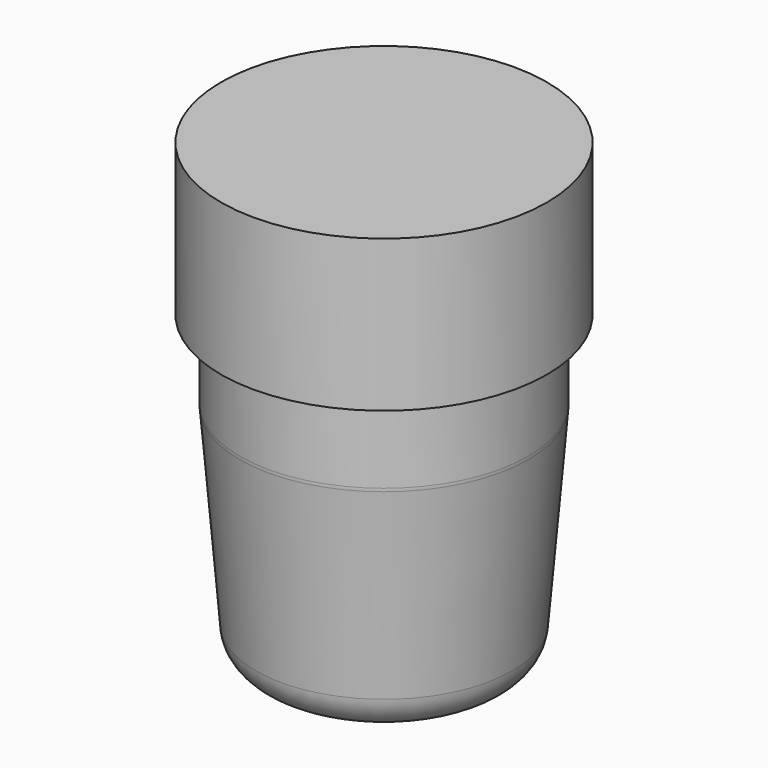
from build123d import *

# Parameters (mm, degrees)
F0_R     = 21.5
F1_DEPTH = 20
F2_R     = 19.0313090647
F3_DEPTH = 0.5
F4_R     = 19.0313090647
F5_DEPTH = 40


# Not quite as in the source:
# - a fillet or chamfer that OpenCascade refuses, or shapes differently, is made with other operations: its cross-section is extruded or revolved along the edge and cut away or added


with BuildPart() as f1:
    # F0 (on Top) → F1 (new body)
    with BuildSketch(Plane.XY):
        Circle(F0_R)
    extrude(amount=F1_DEPTH)

    # F2 (on face) → F3 (join)
    with BuildSketch(Plane(origin=(0, 0, 0), x_dir=(1, 0, 0), z_dir=(0, 0, -1))):
        Circle(F2_R)
    extrude(amount=F3_DEPTH)

    # F4 (on face) → F5 (join)
    with BuildSketch(Plane(origin=(0, 0, -0.5), x_dir=(1, 0, 0), z_dir=(0, 0, -1))):
        Circle(F4_R)
    extrude(amount=F5_DEPTH)

    # F6: chamfer of 2.5 x 30 on 1 edges, made by hand

    # F6_s1 → F6_t2 (revolve, cut)
    with BuildSketch(Plane.XZ):
        Polygon((19.0313090647, -10.5), (16.5313090647, -40.5), (19.0313090647, -40.5), align=None)
    revolve(axis=Axis((0, 0, -40.5), (0, 0, -1)), mode=Mode.SUBTRACT)

    # F7: fillet of radius 5 on 2 edges, made by hand

    # F7_s1 → F7_t2 (revolve, cut)
    with BuildSketch(Plane.XZ):
        with BuildLine():
            ThreePointArc((16.9133734481, -35.9152273993), (15.3161921018, -39.1794114337), (11.9306446569, -40.5))
            Line((11.9306446569, -40.5), (16.5313090647, -40.5))
            Line((16.5313090647, -40.5), (16.9133734481, -35.9152273993))
        make_face()
    revolve(axis=Axis((0, 0, -40.5), (0, 0, -1)), mode=Mode.SUBTRACT)

    # F7_s3 → F7_t4 (revolve, cut)
    with BuildSketch(Plane.XZ):
        with BuildLine():
            ThreePointArc((19.0313090647, -10.2920271064), (19.0269893965, -10.4998203255), (19.0140378559, -10.7072545056))
            Line((19.0140378559, -10.7072545056), (19.0313090647, -10.5))
            Line((19.0313090647, -10.5), (19.0313090647, -10.2920271064))
        make_face()
    revolve(axis=Axis((0, 0, -10.5), (0, 0, -1)), mode=Mode.SUBTRACT)


solid = f1.part
